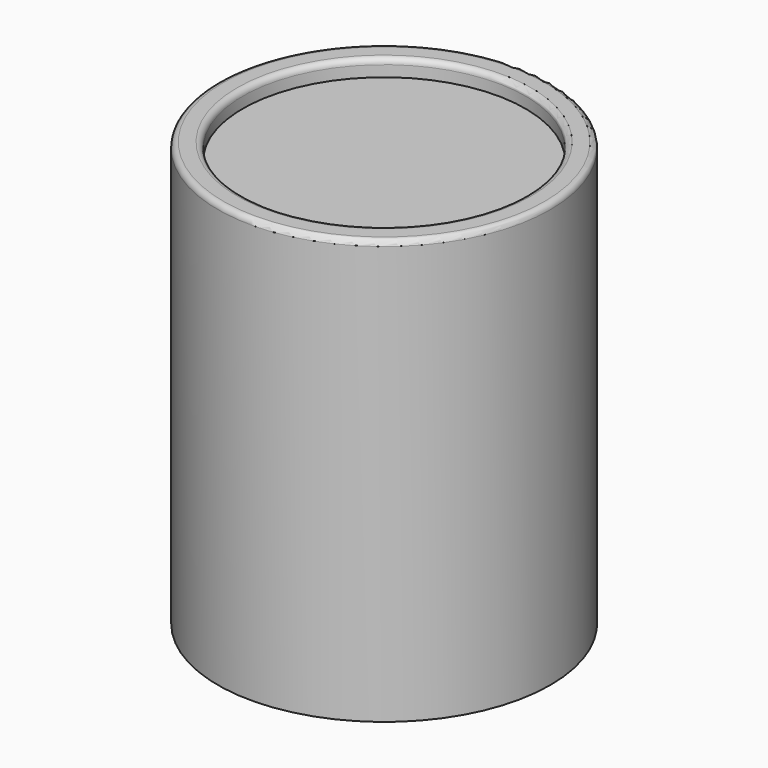
from build123d import *

# Parameters (mm, degrees)
F0_R     = 30
F1_DEPTH = 73
F2_DEPTH = 3.5
F5_D     = 51
F5_DEPTH = 3.5
F5_TIP   = 15.3219457852
F6_R     = 1
F7_T     = -1.3


with BuildPart() as f1:
    # F0 (on Top) → F1 (new body)
    with BuildSketch(Plane.XY):
        Circle(F0_R)
    extrude(amount=F1_DEPTH)

    # F2 (add): a face of the model
    f2_faces = [f1.faces().sort_by_distance(p)[0] for p in [
        (0, 0, 73),
    ]]
    extrude(f2_faces, amount=F2_DEPTH)

    # F5 (one way)
    with BuildSketch(Plane(origin=(0, 0, 73.5), x_dir=(1, 0, 0), z_dir=(0, 0, -1))):
        with Locations((0, 0)):
            Circle(F5_D / 2)
    extrude(amount=-F5_DEPTH, mode=Mode.SUBTRACT)
    with Locations(Plane(origin=(0, 0, 73.5), x_dir=(1, 0, 0), z_dir=(0, 0, -1))):
        with Locations((0, 0)):
            with Locations((0, 0, -(F5_DEPTH + F5_TIP / 2))):  # 118° drill point
                Cone(0, F5_D / 2, F5_TIP, mode=Mode.SUBTRACT)

    # F6
    f6_edges = [f1.edges().sort_by_distance(p)[0] for p in [
        (-30, 0, 76.5),
        (-25.5, 0, 76.5),
    ]]
    fillet(f6_edges, radius=F6_R)

    # F7
    f7_openings = [f1.faces().sort_by_distance(p)[0] for p in [
        (0, 0, 0),
    ]]
    offset(amount=F7_T, openings=f7_openings, kind=Kind.INTERSECTION)


solid = f1.part
